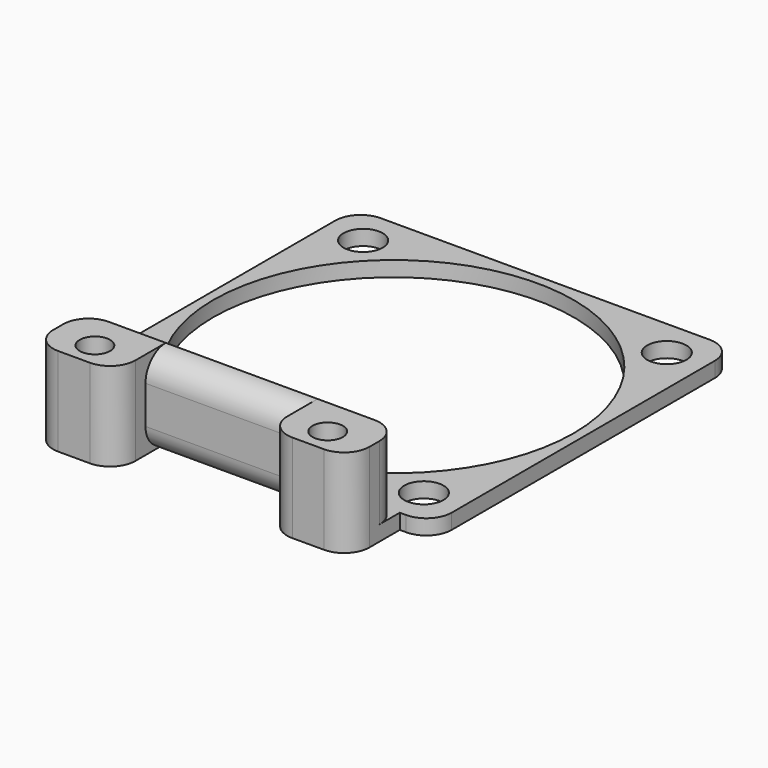
from build123d import *

# Parameters (mm, degrees)
F0_R     = 1.55
F0_R_2   = 14.25
F0_R_3   = 1.2
F0_W     = 12
F0_H     = 2
F1_DEPTH = 1.2
F2_DEPTH = 7
F3_R     = 2
F3_R_2   = 1.99999


# Not quite as in the source:
# - a fillet or chamfer is up to 0.001 mm smaller than in the source, because OpenCascade refuses the exact size


with BuildPart() as f1:
    # F0 (on Top) → F1 (new body)
    with BuildSketch(Plane.XY):
        Polygon((12.5, -15), (15, -15), (15, 15), (-15, 15), (-15, -15), (-12.5, -15), (-6, -15), (6, -15), align=None)
        with Locations((-12, -12)):
            Circle(F0_R, mode=Mode.SUBTRACT)
        with Locations((12, -12)):
            Circle(F0_R, mode=Mode.SUBTRACT)
        with Locations((-12, 12)):
            Circle(F0_R, mode=Mode.SUBTRACT)
        Circle(F0_R_2, mode=Mode.SUBTRACT)
        with Locations((12, 12)):
            Circle(F0_R, mode=Mode.SUBTRACT)
        Polygon((-6, -17), (-6, -15), (-12.5, -15), (-12.5, -20), (-6, -20), align=None)
        with Locations((-9.2, -18)):
            Circle(F0_R_3, mode=Mode.SUBTRACT)
        with Locations((0, -16)):
            Rectangle(F0_W, F0_H)
        Polygon((12.5, -20), (12.5, -15), (6, -15), (6, -17), (6, -20), align=None)
        with Locations((9.2, -18)):
            Circle(F0_R_3, mode=Mode.SUBTRACT)
    extrude(amount=F1_DEPTH)

    # F0 (on Top) → F2 (join)
    with BuildSketch(Plane.XY):
        with Locations((0, -16)):
            Rectangle(F0_W, F0_H)
        Polygon((-6, -17), (-6, -15), (-12.5, -15), (-12.5, -20), (-6, -20), align=None)
        with Locations((-9.2, -18)):
            Circle(F0_R_3, mode=Mode.SUBTRACT)
        Polygon((12.5, -20), (12.5, -15), (6, -15), (6, -17), (6, -20), align=None)
        with Locations((9.2, -18)):
            Circle(F0_R_3, mode=Mode.SUBTRACT)
    extrude(amount=F2_DEPTH)

    # F3 (call 1 of 12: OpenCascade refuses the feature's edges together)
    f3_edges = [f1.edges().sort_by_distance(p)[0] for p in [
        (15, -15, 0.6),
    ]]
    fillet(f3_edges, radius=F3_R)

    # F3#2 (call 2 of 12)
    f3_2_edges = [f1.edges().sort_by_distance(p)[0] for p in [
        (-15, -15, 0.6),
    ]]
    fillet(f3_2_edges, radius=F3_R)

    # F3#3 (call 3 of 12)
    f3_3_edges = [f1.edges().sort_by_distance(p)[0] for p in [
        (-15, 15, 0.6),
    ]]
    fillet(f3_3_edges, radius=F3_R)

    # F3#4 (call 4 of 12)
    f3_4_edges = [f1.edges().sort_by_distance(p)[0] for p in [
        (15, 15, 0.6),
    ]]
    fillet(f3_4_edges, radius=F3_R)

    # F3#5 (call 5 of 12)
    f3_5_edges = [f1.edges().sort_by_distance(p)[0] for p in [
        (-12.5, -20, 3.5),
    ]]
    fillet(f3_5_edges, radius=F3_R)

    # F3#6 (call 6 of 12)
    f3_6_edges = [f1.edges().sort_by_distance(p)[0] for p in [
        (-6, -20, 3.5),
    ]]
    fillet(f3_6_edges, radius=F3_R)

    # F3#7 (call 7 of 12)
    f3_7_edges = [f1.edges().sort_by_distance(p)[0] for p in [
        (6, -20, 3.5),
    ]]
    fillet(f3_7_edges, radius=F3_R)

    # F3#8 (call 8 of 12)
    f3_8_edges = [f1.edges().sort_by_distance(p)[0] for p in [
        (12.5, -20, 3.5),
    ]]
    fillet(f3_8_edges, radius=F3_R)

    # F3#9 (call 9 of 12)
    f3_9_edges = [f1.edges().sort_by_distance(p)[0] for p in [
        (12.5, -15, 4.1),
    ]]
    fillet(f3_9_edges, radius=F3_R)

    # F3#10 (call 10 of 12)
    f3_10_edges = [f1.edges().sort_by_distance(p)[0] for p in [
        (-12.5, -15, 4.1),
    ]]
    fillet(f3_10_edges, radius=F3_R)

    # F3#11 (call 11 of 12) (radius 2 in the source; OpenCascade refuses exactly that, so slightly less here)
    f3_11_edges = [f1.edges().sort_by_distance(p)[0] for p in [
        (0, -17, 7),
    ]]
    fillet(f3_11_edges, radius=F3_R_2)

    # F3#12 (call 12 of 12)
    f3_12_edges = [f1.edges().sort_by_distance(p)[0] for p in [
        (0, -17, 0),
    ]]
    fillet(f3_12_edges, radius=F3_R)


solid = f1.part
